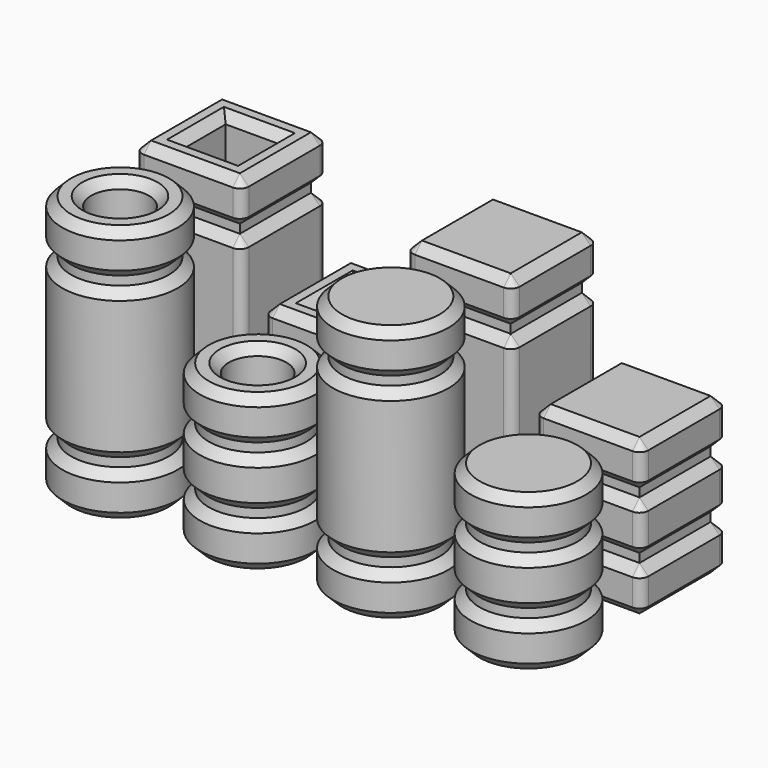
from build123d import *

# Parameters (mm, degrees)
F1_DEPTH    = 10
F0_R        = 13
F0_R_2      = 6.5
F0_W        = 12
F0_H        = 12
F2_W        = 20
F2_H        = 20
F2_W_2      = 12
F2_H_2      = 12
F3_DEPTH    = 48
F2_R        = 11
F2_R_2      = 6.5
F4_DEPTH    = 25
F5_START    = 12
F5_DEPTH    = 34
F6_START    = 12
F6_DEPTH    = 11
F7_START    = 2
F5_FACE_W   = 20
F5_FACE_H   = 20
F7_DEPTH    = 10
F5_FACE_R   = 13
F5_FACE_R_2 = 11
F6_FACE_W   = 20
F6_FACE_H   = 20
F6_FACE_R   = 13
F6_FACE_R_2 = 11
F8_SIZE     = 1.99999
F8_2_SIZE   = 1.99999
F8_3_SIZE   = 1.99999
F8_4_SIZE   = 1.99999
F8_5_SIZE   = 1.99999
F8_6_SIZE   = 1.99999
F8_7_SIZE   = 1.99999
F8_8_SIZE   = 1.99999


# Not quite as in the source:
# - a fillet or chamfer is up to 0.001 mm smaller than in the source, because OpenCascade refuses the exact size


with BuildPart() as f1:
    # F0 (on Top) → F1 (new body)
    with BuildSketch(Plane.XY):
        with BuildLine():
            ThreePointArc((28, 24.5), (27.4142135624, 25.9142135624), (26, 26.5))
            Line((26, 26.5), (6, 26.5))
            ThreePointArc((6, 26.5), (4.5857864376, 25.9142135624), (4, 24.5))
            Line((4, 24.5), (4, 4.5))
            ThreePointArc((4, 4.5), (4.5857864376, 3.0857864376), (6, 2.5))
            Line((6, 2.5), (26, 2.5))
            ThreePointArc((26, 2.5), (27.4142135624, 3.0857864376), (28, 4.5))
            Line((28, 4.5), (28, 24.5))
        make_face()
    extrude(amount=F1_DEPTH)

    # F2 (on face) → F3, piece 4 (join)
    with BuildSketch(Plane.XY.offset(10)):
        with Locations((16, 14.5)):
            Rectangle(F2_W, F2_H)
    extrude(amount=F3_DEPTH)

    # F0 (on Top) → F5, piece 4 (join)
    with BuildSketch(Plane.XY.offset(F5_START)):
        with BuildLine():
            ThreePointArc((28, 24.5), (27.4142135624, 25.9142135624), (26, 26.5))
            Line((26, 26.5), (6, 26.5))
            ThreePointArc((6, 26.5), (4.5857864376, 25.9142135624), (4, 24.5))
            Line((4, 24.5), (4, 4.5))
            ThreePointArc((4, 4.5), (4.5857864376, 3.0857864376), (6, 2.5))
            Line((6, 2.5), (26, 2.5))
            ThreePointArc((26, 2.5), (27.4142135624, 3.0857864376), (28, 4.5))
            Line((28, 4.5), (28, 24.5))
        make_face()
    extrude(amount=F5_DEPTH)

    # F5_face (on face) → F7, piece 5 (join)
    with BuildSketch(Plane(origin=(-45, 14.5, 46), x_dir=(1, 0, 0), z_dir=(0, 0, 1)).offset(F7_START)):
        with BuildLine():
            ThreePointArc((73, 10), (72.4142135624, 11.4142135624), (71, 12))
            Line((71, 12), (51, 12))
            ThreePointArc((51, 12), (49.5857864376, 11.4142135624), (49, 10))
            Line((49, 10), (49, -10))
            ThreePointArc((49, -10), (49.5857864376, -11.4142135624), (51, -12))
            Line((51, -12), (71, -12))
            ThreePointArc((71, -12), (72.4142135624, -11.4142135624), (73, -10))
            Line((73, -10), (73, 10))
        make_face()
        with Locations((61, 0)):
            Rectangle(F5_FACE_W, F5_FACE_H, mode=Mode.SUBTRACT)
    extrude(amount=F7_DEPTH)

    # F8#5 (size 2 in the source; OpenCascade refuses exactly that, so slightly less here)
    f8_5_edges = [f1.edges().sort_by_distance(p)[0] for p in [
        (27.414214, 25.914214, 0),
        (16, 26.5, 0),
        (4.585786, 25.914214, 0),
        (4, 14.5, 0),
        (4.585786, 3.085786, 0),
        (16, 2.5, 0),
        (27.414214, 3.085786, 0),
        (28, 14.5, 0),
        (16, 26.5, 10),
        (28, 14.5, 10),
        (16, 26.5, 12),
        (28, 14.5, 12),
        (4, 14.5, 10),
        (4, 14.5, 12),
        (16, 2.5, 10),
        (16, 2.5, 12),
        (4, 14.5, 46),
        (4, 14.5, 48),
        (16, 2.5, 48),
        (16, 2.5, 46),
        (16, 26.5, 46),
        (16, 26.5, 48),
        (28, 14.5, 46),
        (28, 14.5, 48),
        (27.414214, 3.085786, 58),
        (28, 14.5, 58),
        (27.414214, 25.914214, 58),
        (16, 26.5, 58),
        (4.585786, 25.914214, 58),
        (4, 14.5, 58),
        (4.585786, 3.085786, 58),
        (16, 2.5, 58),
    ]]
    chamfer(f8_5_edges, length=F8_5_SIZE)


with BuildPart() as f1b:
    # F0 (on Top) → F1, piece 2 (new body)
    with BuildSketch(Plane.XY):
        with Locations((15, -15.5)):
            Circle(F0_R)
    extrude(amount=F1_DEPTH)

    # F2 (on face) → F3, piece 3 (join)
    with BuildSketch(Plane.XY.offset(10)):
        with Locations((15, -15.5)):
            Circle(F2_R)
    extrude(amount=F3_DEPTH)

    # F0 (on Top) → F5, piece 3 (join)
    with BuildSketch(Plane.XY.offset(F5_START)):
        with Locations((15, -15.5)):
            Circle(F0_R)
    extrude(amount=F5_DEPTH)

    # F5_face (on face) → F7, piece 6 (join)
    with BuildSketch(Plane(origin=(-45, 14.5, 46), x_dir=(1, 0, 0), z_dir=(0, 0, 1)).offset(F7_START)):
        with Locations((60, -30)):
            Circle(F5_FACE_R)
        with Locations((60, -30)):
            Circle(F5_FACE_R_2, mode=Mode.SUBTRACT)
    extrude(amount=F7_DEPTH)

    # F8#6 (size 2 in the source; OpenCascade refuses exactly that, so slightly less here)
    f8_6_edges = [f1b.edges().sort_by_distance(p)[0] for p in [
        (2, -15.5, 0),
        (28, -15.5, 5),
        (2, -15.5, 10),
        (2, -15.5, 12),
        (2, -15.5, 46),
        (2, -15.5, 48),
        (2, -15.5, 58),
    ]]
    chamfer(f8_6_edges, length=F8_6_SIZE)


with BuildPart() as f1c:
    # F0 (on Top) → F1, piece 3 (new body)
    with BuildSketch(Plane.XY):
        with Locations((-46, -15.5)):
            Circle(F0_R)
        with Locations((-46, -15.5)):
            Circle(F0_R_2, mode=Mode.SUBTRACT)
    extrude(amount=F1_DEPTH)

    # F2 (on face) → F3, piece 2 (join)
    with BuildSketch(Plane.XY.offset(10)):
        with Locations((-46, -15.5)):
            Circle(F2_R)
        with Locations((-46, -15.5)):
            Circle(F2_R_2, mode=Mode.SUBTRACT)
    extrude(amount=F3_DEPTH)

    # F0 (on Top) → F5, piece 2 (join)
    with BuildSketch(Plane.XY.offset(F5_START)):
        with Locations((-46, -15.5)):
            Circle(F0_R)
        with Locations((-46, -15.5)):
            Circle(F0_R_2, mode=Mode.SUBTRACT)
    extrude(amount=F5_DEPTH)

    # F5_face (on face) → F7, piece 2 (join)
    with BuildSketch(Plane(origin=(-45, 14.5, 46), x_dir=(1, 0, 0), z_dir=(0, 0, 1)).offset(F7_START)):
        with Locations((-1, -30)):
            Circle(F5_FACE_R)
        with Locations((-1, -30)):
            Circle(F5_FACE_R_2, mode=Mode.SUBTRACT)
    extrude(amount=F7_DEPTH)

    # F8#2 (size 2 in the source; OpenCascade refuses exactly that, so slightly less here)
    f8_2_edges = [f1c.edges().sort_by_distance(p)[0] for p in [
        (-59, -15.5, 0),
        (-52.5, -15.5, 0),
        (-59, -15.5, 10),
        (-59, -15.5, 12),
        (-59, -15.5, 46),
        (-59, -15.5, 48),
        (-52.5, -15.5, 58),
        (-59, -15.5, 58),
    ]]
    chamfer(f8_2_edges, length=F8_2_SIZE)


with BuildPart() as f1d:
    # F0 (on Top) → F1, piece 4 (new body)
    with BuildSketch(Plane.XY):
        with BuildLine():
            ThreePointArc((-6, 2.5), (-4.5857864376, 3.0857864376), (-4, 4.5))
            Line((-4, 4.5), (-4, 24.5))
            ThreePointArc((-4, 24.5), (-4.5857864376, 25.9142135624), (-6, 26.5))
            Line((-6, 26.5), (-26, 26.5))
            ThreePointArc((-26, 26.5), (-27.4142135624, 25.9142135624), (-28, 24.5))
            Line((-28, 24.5), (-28, 4.5))
            ThreePointArc((-28, 4.5), (-27.4142135624, 3.0857864376), (-26, 2.5))
            Line((-26, 2.5), (-6, 2.5))
        make_face()
        with Locations((-16, 14.5)):
            Rectangle(F0_W, F0_H, mode=Mode.SUBTRACT)
    extrude(amount=F1_DEPTH)

    # F2 (on face) → F4 (join)
    with BuildSketch(Plane.XY.offset(10)):
        with Locations((-16, 14.5)):
            Rectangle(F2_W, F2_H)
        with Locations((-16, 14.5)):
            Rectangle(F2_W_2, F2_H_2, mode=Mode.SUBTRACT)
    extrude(amount=F4_DEPTH)

    # F0 (on Top) → F6 (join)
    with BuildSketch(Plane.XY.offset(F6_START)):
        with BuildLine():
            ThreePointArc((-6, 2.5), (-4.5857864376, 3.0857864376), (-4, 4.5))
            Line((-4, 4.5), (-4, 24.5))
            ThreePointArc((-4, 24.5), (-4.5857864376, 25.9142135624), (-6, 26.5))
            Line((-6, 26.5), (-26, 26.5))
            ThreePointArc((-26, 26.5), (-27.4142135624, 25.9142135624), (-28, 24.5))
            Line((-28, 24.5), (-28, 4.5))
            ThreePointArc((-28, 4.5), (-27.4142135624, 3.0857864376), (-26, 2.5))
            Line((-26, 2.5), (-6, 2.5))
        make_face()
        with Locations((-16, 14.5)):
            Rectangle(F0_W, F0_H, mode=Mode.SUBTRACT)
    extrude(amount=F6_DEPTH)

    # F6_face (on face) → F7, piece 3 (join)
    with BuildSketch(Plane(origin=(-16, 14.5, 23), x_dir=(1, 0, 0), z_dir=(0, 0, 1)).offset(F7_START)):
        with BuildLine():
            ThreePointArc((10, -12), (11.4142135624, -11.4142135624), (12, -10))
            Line((12, -10), (12, 10))
            ThreePointArc((12, 10), (11.4142135624, 11.4142135624), (10, 12))
            Line((10, 12), (-10, 12))
            ThreePointArc((-10, 12), (-11.4142135624, 11.4142135624), (-12, 10))
            Line((-12, 10), (-12, -10))
            ThreePointArc((-12, -10), (-11.4142135624, -11.4142135624), (-10, -12))
            Line((-10, -12), (10, -12))
        make_face()
        Rectangle(F6_FACE_W, F6_FACE_H, mode=Mode.SUBTRACT)
    extrude(amount=F7_DEPTH)

    # F8#3 (size 2 in the source; OpenCascade refuses exactly that, so slightly less here)
    f8_3_edges = [f1d.edges().sort_by_distance(p)[0] for p in [
        (-4.585786, 3.085786, 0),
        (-4, 14.5, 0),
        (-4.585786, 25.914214, 0),
        (-16, 26.5, 0),
        (-27.414214, 25.914214, 0),
        (-28, 14.5, 0),
        (-27.414214, 3.085786, 0),
        (-16, 2.5, 0),
        (-22, 14.5, 0),
        (-16, 20.5, 0),
        (-10, 14.5, 0),
        (-16, 8.5, 0),
        (-16, 2.5, 10),
        (-16, 2.5, 12),
        (-28, 14.5, 10),
        (-28, 14.5, 12),
        (-4, 14.5, 12),
        (-4, 14.5, 10),
        (-16, 26.5, 12),
        (-16, 26.5, 10),
        (-16, 26.5, 23),
        (-16, 26.5, 25),
        (-4, 14.5, 25),
        (-4, 14.5, 23),
        (-16, 2.5, 25),
        (-16, 2.5, 23),
        (-28, 14.5, 25),
        (-28, 14.5, 23),
        (-16, 8.5, 35),
        (-22, 14.5, 35),
        (-16, 20.5, 35),
        (-10, 14.5, 35),
        (-4.585786, 3.085786, 35),
        (-4, 14.5, 35),
        (-4.585786, 25.914214, 35),
        (-16, 26.5, 35),
        (-27.414214, 25.914214, 35),
        (-28, 14.5, 35),
        (-27.414214, 3.085786, 35),
        (-16, 2.5, 35),
    ]]
    chamfer(f8_3_edges, length=F8_3_SIZE)


with BuildPart() as f1e:
    # F0 (on Top) → F1, piece 5 (new body)
    with BuildSketch(Plane.XY):
        with Locations((-15, -15.5)):
            Circle(F0_R)
        with Locations((-15, -15.5)):
            Circle(F0_R_2, mode=Mode.SUBTRACT)
    extrude(amount=F1_DEPTH)

    # F2 (on face) → F4, piece 2 (join)
    with BuildSketch(Plane.XY.offset(10)):
        with Locations((-15, -15.5)):
            Circle(F2_R)
        with Locations((-15, -15.5)):
            Circle(F2_R_2, mode=Mode.SUBTRACT)
    extrude(amount=F4_DEPTH)

    # F0 (on Top) → F6, piece 2 (join)
    with BuildSketch(Plane.XY.offset(F6_START)):
        with Locations((-15, -15.5)):
            Circle(F0_R)
        with Locations((-15, -15.5)):
            Circle(F0_R_2, mode=Mode.SUBTRACT)
    extrude(amount=F6_DEPTH)

    # F6_face (on face) → F7, piece 4 (join)
    with BuildSketch(Plane(origin=(-16, 14.5, 23), x_dir=(1, 0, 0), z_dir=(0, 0, 1)).offset(F7_START)):
        with Locations((1, -30)):
            Circle(F6_FACE_R)
        with Locations((1, -30)):
            Circle(F6_FACE_R_2, mode=Mode.SUBTRACT)
    extrude(amount=F7_DEPTH)

    # F8#4 (size 2 in the source; OpenCascade refuses exactly that, so slightly less here)
    f8_4_edges = [f1e.edges().sort_by_distance(p)[0] for p in [
        (-28, -15.5, 0),
        (-21.5, -15.5, 0),
        (-28, -15.5, 10),
        (-28, -15.5, 12),
        (-28, -15.5, 23),
        (-28, -15.5, 25),
        (-21.5, -15.5, 35),
        (-28, -15.5, 35),
    ]]
    chamfer(f8_4_edges, length=F8_4_SIZE)


with BuildPart() as f1f:
    # F0 (on Top) → F1, piece 6 (new body)
    with BuildSketch(Plane.XY):
        with BuildLine():
            ThreePointArc((33, 4.5), (33.5857864376, 3.0857864376), (35, 2.5))
            Line((35, 2.5), (55, 2.5))
            ThreePointArc((55, 2.5), (56.4142135624, 3.0857864376), (57, 4.5))
            Line((57, 4.5), (57, 24.5))
            ThreePointArc((57, 24.5), (56.4142135624, 25.9142135624), (55, 26.5))
            Line((55, 26.5), (35, 26.5))
            ThreePointArc((35, 26.5), (33.5857864376, 25.9142135624), (33, 24.5))
            Line((33, 24.5), (33, 4.5))
        make_face()
    extrude(amount=F1_DEPTH)

    # F2 (on face) → F4, piece 3 (join)
    with BuildSketch(Plane.XY.offset(10)):
        with Locations((45, 14.5)):
            Rectangle(F2_W, F2_H)
    extrude(amount=F4_DEPTH)

    # F0 (on Top) → F6, piece 4 (join)
    with BuildSketch(Plane.XY.offset(F6_START)):
        with BuildLine():
            ThreePointArc((33, 4.5), (33.5857864376, 3.0857864376), (35, 2.5))
            Line((35, 2.5), (55, 2.5))
            ThreePointArc((55, 2.5), (56.4142135624, 3.0857864376), (57, 4.5))
            Line((57, 4.5), (57, 24.5))
            ThreePointArc((57, 24.5), (56.4142135624, 25.9142135624), (55, 26.5))
            Line((55, 26.5), (35, 26.5))
            ThreePointArc((35, 26.5), (33.5857864376, 25.9142135624), (33, 24.5))
            Line((33, 24.5), (33, 4.5))
        make_face()
    extrude(amount=F6_DEPTH)

    # F6_face (on face) → F7, piece 7 (join)
    with BuildSketch(Plane(origin=(-16, 14.5, 23), x_dir=(1, 0, 0), z_dir=(0, 0, 1)).offset(F7_START)):
        with BuildLine():
            ThreePointArc((49, -10), (49.5857864376, -11.4142135624), (51, -12))
            Line((51, -12), (71, -12))
            ThreePointArc((71, -12), (72.4142135624, -11.4142135624), (73, -10))
            Line((73, -10), (73, 10))
            ThreePointArc((73, 10), (72.4142135624, 11.4142135624), (71, 12))
            Line((71, 12), (51, 12))
            ThreePointArc((51, 12), (49.5857864376, 11.4142135624), (49, 10))
            Line((49, 10), (49, -10))
        make_face()
        with Locations((61, 0)):
            Rectangle(F6_FACE_W, F6_FACE_H, mode=Mode.SUBTRACT)
    extrude(amount=F7_DEPTH)

    # F8#7 (size 2 in the source; OpenCascade refuses exactly that, so slightly less here)
    f8_7_edges = [f1f.edges().sort_by_distance(p)[0] for p in [
        (33.585786, 3.085786, 0),
        (45, 2.5, 0),
        (56.414214, 3.085786, 0),
        (57, 14.5, 0),
        (56.414214, 25.914214, 0),
        (45, 26.5, 0),
        (33.585786, 25.914214, 0),
        (33, 14.5, 0),
        (45, 26.5, 10),
        (45, 26.5, 12),
        (57, 14.5, 10),
        (57, 14.5, 12),
        (33, 14.5, 10),
        (33, 14.5, 12),
        (45, 2.5, 12),
        (45, 2.5, 10),
        (45, 2.5, 25),
        (45, 2.5, 23),
        (57, 14.5, 25),
        (57, 14.5, 23),
        (45, 26.5, 25),
        (45, 26.5, 23),
        (33, 14.5, 23),
        (33, 14.5, 25),
        (33.585786, 3.085786, 35),
        (45, 2.5, 35),
        (56.414214, 3.085786, 35),
        (57, 14.5, 35),
        (56.414214, 25.914214, 35),
        (45, 26.5, 35),
        (33.585786, 25.914214, 35),
        (33, 14.5, 35),
    ]]
    chamfer(f8_7_edges, length=F8_7_SIZE)


with BuildPart() as f1g:
    # F0 (on Top) → F1, piece 7 (new body)
    with BuildSketch(Plane.XY):
        with Locations((46, -15.5)):
            Circle(F0_R)
    extrude(amount=F1_DEPTH)

    # F2 (on face) → F4, piece 4 (join)
    with BuildSketch(Plane.XY.offset(10)):
        with Locations((46, -15.5)):
            Circle(F2_R)
    extrude(amount=F4_DEPTH)

    # F0 (on Top) → F6, piece 3 (join)
    with BuildSketch(Plane.XY.offset(F6_START)):
        with Locations((46, -15.5)):
            Circle(F0_R)
    extrude(amount=F6_DEPTH)

    # F6_face (on face) → F7, piece 8 (join)
    with BuildSketch(Plane(origin=(-16, 14.5, 23), x_dir=(1, 0, 0), z_dir=(0, 0, 1)).offset(F7_START)):
        with Locations((62, -30)):
            Circle(F6_FACE_R)
        with Locations((62, -30)):
            Circle(F6_FACE_R_2, mode=Mode.SUBTRACT)
    extrude(amount=F7_DEPTH)

    # F8#8 (size 2 in the source; OpenCascade refuses exactly that, so slightly less here)
    f8_8_edges = [f1g.edges().sort_by_distance(p)[0] for p in [
        (33, -15.5, 0),
        (33, -15.5, 10),
        (33, -15.5, 12),
        (33, -15.5, 23),
        (33, -15.5, 25),
        (33, -15.5, 35),
    ]]
    chamfer(f8_8_edges, length=F8_8_SIZE)


with BuildPart() as f1h:
    # F0 (on Top) → F1, piece 8 (new body)
    with BuildSketch(Plane.XY):
        with BuildLine():
            Line((-55, 2.5), (-35, 2.5))
            ThreePointArc((-35, 2.5), (-33.5857864376, 3.0857864376), (-33, 4.5))
            Line((-33, 4.5), (-33, 24.5))
            ThreePointArc((-33, 24.5), (-33.5857864376, 25.9142135624), (-35, 26.5))
            Line((-35, 26.5), (-55, 26.5))
            ThreePointArc((-55, 26.5), (-56.4142135624, 25.9142135624), (-57, 24.5))
            Line((-57, 24.5), (-57, 4.5))
            ThreePointArc((-57, 4.5), (-56.4142135624, 3.0857864376), (-55, 2.5))
        make_face()
        with Locations((-45, 14.5)):
            Rectangle(F0_W, F0_H, mode=Mode.SUBTRACT)
    extrude(amount=F1_DEPTH)

    # F2 (on face) → F3 (join)
    with BuildSketch(Plane.XY.offset(10)):
        with Locations((-45, 14.5)):
            Rectangle(F2_W, F2_H)
        with Locations((-45, 14.5)):
            Rectangle(F2_W_2, F2_H_2, mode=Mode.SUBTRACT)
    extrude(amount=F3_DEPTH)

    # F0 (on Top) → F5 (join)
    with BuildSketch(Plane.XY.offset(F5_START)):
        with BuildLine():
            Line((-55, 2.5), (-35, 2.5))
            ThreePointArc((-35, 2.5), (-33.5857864376, 3.0857864376), (-33, 4.5))
            Line((-33, 4.5), (-33, 24.5))
            ThreePointArc((-33, 24.5), (-33.5857864376, 25.9142135624), (-35, 26.5))
            Line((-35, 26.5), (-55, 26.5))
            ThreePointArc((-55, 26.5), (-56.4142135624, 25.9142135624), (-57, 24.5))
            Line((-57, 24.5), (-57, 4.5))
            ThreePointArc((-57, 4.5), (-56.4142135624, 3.0857864376), (-55, 2.5))
        make_face()
        with Locations((-45, 14.5)):
            Rectangle(F0_W, F0_H, mode=Mode.SUBTRACT)
    extrude(amount=F5_DEPTH)

    # F5_face (on face) → F7 (join)
    with BuildSketch(Plane(origin=(-45, 14.5, 46), x_dir=(1, 0, 0), z_dir=(0, 0, 1)).offset(F7_START)):
        with BuildLine():
            Line((-10, -12), (10, -12))
            ThreePointArc((10, -12), (11.4142135624, -11.4142135624), (12, -10))
            Line((12, -10), (12, 10))
            ThreePointArc((12, 10), (11.4142135624, 11.4142135624), (10, 12))
            Line((10, 12), (-10, 12))
            ThreePointArc((-10, 12), (-11.4142135624, 11.4142135624), (-12, 10))
            Line((-12, 10), (-12, -10))
            ThreePointArc((-12, -10), (-11.4142135624, -11.4142135624), (-10, -12))
        make_face()
        Rectangle(F5_FACE_W, F5_FACE_H, mode=Mode.SUBTRACT)
    extrude(amount=F7_DEPTH)

    # F8 (size 2 in the source; OpenCascade refuses exactly that, so slightly less here)
    f8_edges = [f1h.edges().sort_by_distance(p)[0] for p in [
        (-45, 26.5, 0),
        (-57, 14.5, 0),
        (-45, 2.5, 0),
        (-33, 14.5, 0),
        (-39, 14.5, 0),
        (-45, 8.5, 0),
        (-51, 14.5, 0),
        (-45, 20.5, 0),
        (-57, 14.5, 10),
        (-45, 26.5, 10),
        (-45, 26.5, 12),
        (-57, 14.5, 12),
        (-45, 2.5, 10),
        (-45, 2.5, 12),
        (-33, 14.5, 10),
        (-33, 14.5, 12),
        (-57, 14.5, 46),
        (-57, 14.5, 48),
        (-45, 2.5, 46),
        (-45, 2.5, 48),
        (-45, 26.5, 46),
        (-45, 26.5, 48),
        (-33, 14.5, 46),
        (-33, 14.5, 48),
        (-45, 8.5, 58),
        (-51, 14.5, 58),
        (-45, 20.5, 58),
        (-39, 14.5, 58),
        (-45, 2.5, 58),
        (-33.585786, 3.085786, 58),
        (-33, 14.5, 58),
        (-33.585786, 25.914214, 58),
        (-45, 26.5, 58),
        (-56.414214, 25.914214, 58),
        (-57, 14.5, 58),
        (-56.414214, 3.085786, 58),
    ]]
    chamfer(f8_edges, length=F8_SIZE)


solid = Compound([f1.part, f1b.part, f1c.part, f1d.part, f1e.part, f1f.part, f1g.part, f1h.part])
